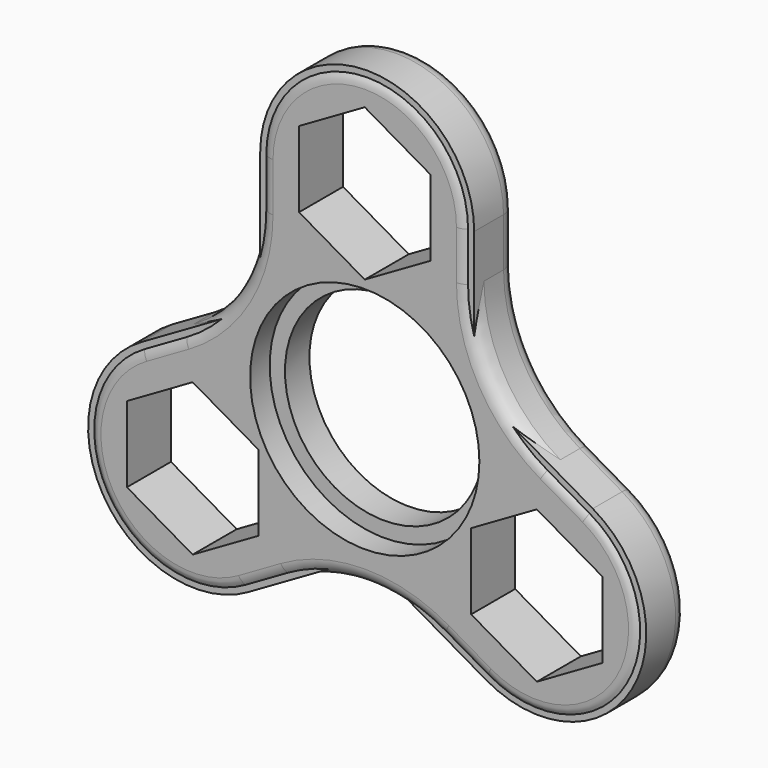
from build123d import *

# Parameters (mm, degrees)
F0_R     = 13
F1_DEPTH = 3.6
F2_R     = 20
F3_R     = 2
F4_R     = 2
F5_DEPTH = 3.2
F6_R     = 15
F7_DEPTH = 3.2


# Not quite as in the source:
# - a feature names something its author has since deleted; it is built from what else it names


with BuildPart() as f1:
    # F0 (on Front) → F1 (new body, symmetric)
    with BuildSketch(Plane.XZ):
        with BuildLine():
            Line((14, 8.0829037687), (14, 26))
            ThreePointArc((14, 26), (0, 40), (-14, 26))
            Line((-14, 26), (-14, 8.0829037687))
            Line((-14, 8.0829037687), (-29.5166604984, -0.875644347))
            ThreePointArc((-29.5166604984, -0.875644347), (-34.6410161514, -20), (-15.5166604984, -25.124355653))
            Line((-15.5166604984, -25.124355653), (0, -16.1658075373))
            Line((0, -16.1658075373), (15.5166604984, -25.124355653))
            ThreePointArc((15.5166604984, -25.124355653), (34.6410161514, -20), (29.5166604984, -0.875644347))
            Line((29.5166604984, -0.875644347), (14, 8.0829037687))
        make_face()
        Polygon((-22.5166604984, -22.9304246301), (-31.1166604984, -17.965212315), (-31.1166604984, -8.034787685), (-22.5166604984, -3.0695753699), (-13.9166604984, -8.034787685), (-13.9166604984, -17.965212315), align=None, mode=Mode.SUBTRACT)
        Polygon((31.1166604984, -8.034787685), (31.1166604984, -17.965212315), (22.5166604984, -22.9304246301), (13.9166604984, -17.965212315), (13.9166604984, -8.034787685), (22.5166604984, -3.0695753699), align=None, mode=Mode.SUBTRACT)
        Circle(F0_R, mode=Mode.SUBTRACT)
        Polygon((0, 35.9304246301), (8.6, 30.965212315), (8.6, 21.034787685), (0, 16.0695753699), (-8.6, 21.034787685), (-8.6, 30.965212315), align=None, mode=Mode.SUBTRACT)
    extrude(amount=F1_DEPTH, both=True)

    # F2
    f2_edges = [f1.edges().sort_by_distance(p)[0] for p in [
        (0, 0, -16.165808),
        (14, 0, 8.082904),
        (-14, 0, 8.082904),
    ]]
    fillet(f2_edges, radius=F2_R)

    # F3
    f3_edges = [f1.edges().sort_by_distance(p)[0] for p in [
        (-14, -3.6, 22.814955),
    ]]
    fillet(f3_edges, radius=F3_R)

    # F4
    f4_edges = [f1.edges().sort_by_distance(p)[0] for p in [
        (0, 3.6, 40),
        (26.75833, 3.6, 0.716878),
        (16.679492, 3.6, 9.629909),
        (34.641016, 3.6, -20),
        (14, 3.6, 22.814955),
        (12.75833, 3.6, -23.531833),
        (0, 3.6, -19.259818),
        (-14, 3.6, 22.814955),
        (-12.75833, 3.6, -23.531833),
        (-16.679492, 3.6, 9.629909),
        (-34.641016, 3.6, -20),
        (-26.75833, 3.6, 0.716878),
    ]]
    fillet(f4_edges, radius=F4_R)

    # F0 (on Front) → F5 (join)
    with BuildSketch(Plane.XZ):
        with BuildLine():
            Line((14, 8.0829037687), (14, 26))
            ThreePointArc((14, 26), (0, 40), (-14, 26))
            Line((-14, 26), (-14, 8.0829037687))
            Line((-14, 8.0829037687), (-29.5166604984, -0.875644347))
            ThreePointArc((-29.5166604984, -0.875644347), (-34.6410161514, -20), (-15.5166604984, -25.124355653))
            Line((-15.5166604984, -25.124355653), (0, -16.1658075373))
            Line((0, -16.1658075373), (15.5166604984, -25.124355653))
            ThreePointArc((15.5166604984, -25.124355653), (34.6410161514, -20), (29.5166604984, -0.875644347))
            Line((29.5166604984, -0.875644347), (14, 8.0829037687))
        make_face()
        Polygon((-22.5166604984, -22.9304246301), (-31.1166604984, -17.965212315), (-31.1166604984, -8.034787685), (-22.5166604984, -3.0695753699), (-13.9166604984, -8.034787685), (-13.9166604984, -17.965212315), align=None, mode=Mode.SUBTRACT)
        Polygon((31.1166604984, -8.034787685), (31.1166604984, -17.965212315), (22.5166604984, -22.9304246301), (13.9166604984, -17.965212315), (13.9166604984, -8.034787685), (22.5166604984, -3.0695753699), align=None, mode=Mode.SUBTRACT)
        Circle(F0_R, mode=Mode.SUBTRACT)
        Polygon((0, 35.9304246301), (8.6, 30.965212315), (8.6, 21.034787685), (0, 16.0695753699), (-8.6, 21.034787685), (-8.6, 30.965212315), align=None, mode=Mode.SUBTRACT)
    extrude(amount=F5_DEPTH)

    # F6 (on face) → F7 (cut)
    with BuildSketch(Plane.XZ.offset(3.6)):
        Circle(F6_R)
    extrude(amount=-F7_DEPTH, mode=Mode.SUBTRACT)


solid = f1.part
